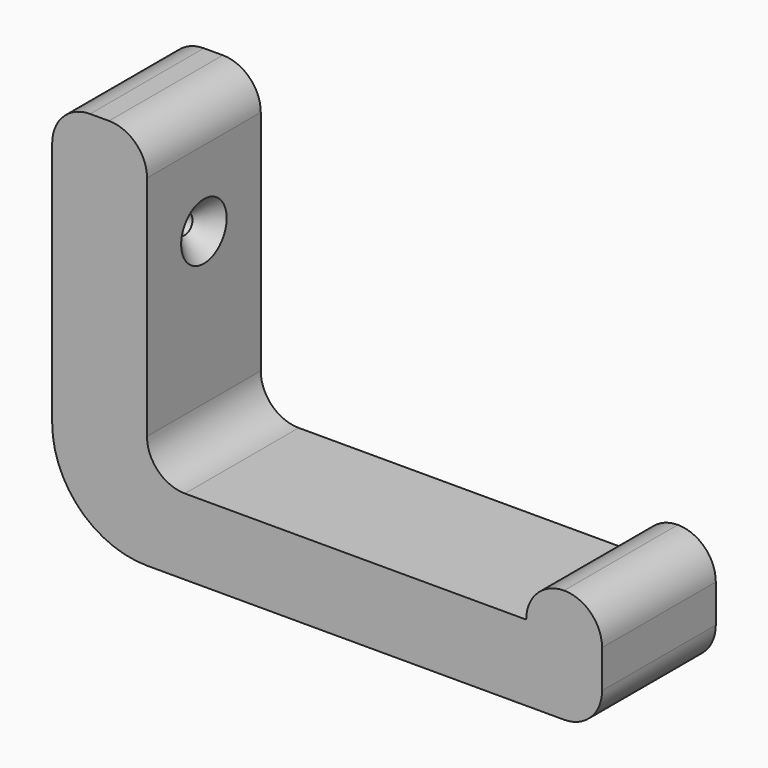
from build123d import *

# Parameters (mm, degrees)
F0_W           = 40
F0_H           = 8
F1_DEPTH       = 15
F2_R           = 3.99999
F3_R           = 10
F5_D           = 2
F5_CSINK_D     = 6
F5_CSINK_ANGLE = 90


# Not quite as in the source:
# - a fillet or chamfer is up to 0.001 mm smaller than in the source, because OpenCascade refuses the exact size


with BuildPart() as f1:
    # F0 (on Front) → F1 (new body)
    with BuildSketch(Plane.XZ):
        Polygon((-20, -4), (-20, 4), (-20, 36), (-30, 36), (-30, -4), align=None)
        Rectangle(F0_W, F0_H)
        Polygon((20, 8), (20, 4), (20, -4), (28, -4), (28, 8), align=None)
    extrude(amount=F1_DEPTH)

    # F2 (radius 4 in the source; OpenCascade refuses exactly that, so slightly less here)
    f2_edges = [f1.edges().sort_by_distance(p)[0] for p in [
        (-20, -7.5, 4),
        (20, -7.5, 8),
        (28, -7.5, 8),
        (28, -7.5, -4),
        (-20, -7.5, 36),
        (-30, -7.5, 36),
    ]]
    fillet(f2_edges, radius=F2_R)

    # F3
    f3_edges = [f1.edges().sort_by_distance(p)[0] for p in [
        (-30, -7.5, -4),
    ]]
    fillet(f3_edges, radius=F3_R)

    # F5 (through all)
    with Locations(Plane.YZ.offset(-20)):
        with Locations((-7.5, 24)):
            CounterSinkHole(F5_D / 2, F5_CSINK_D / 2, counter_sink_angle=F5_CSINK_ANGLE)


solid = f1.part
